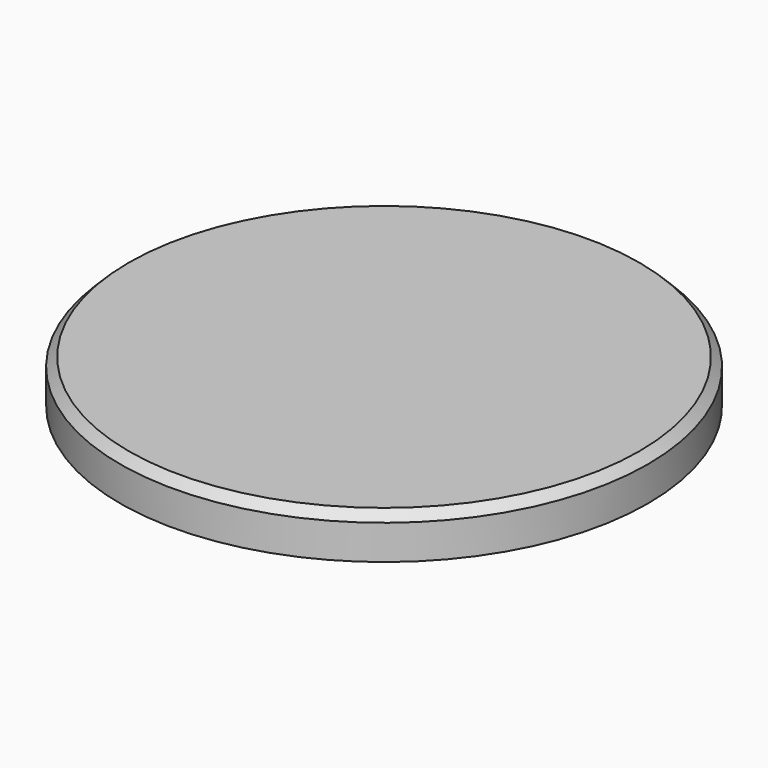
from build123d import *

# Parameters (mm, degrees)
F0_R     = 30.5456119657
F1_DEPTH = 5
F2_SIZE  = 1


# Not quite as in the source:
# - the program builds the solid bodies; features that only make, move or delete a surface that nothing else refers to are left out


with BuildPart() as f1:
    # F0 (on Top) → F1 (new body)
    with BuildSketch(Plane.XY):
        Circle(F0_R)
    extrude(amount=F1_DEPTH)

    # F2
    f2_edges = [f1.edges().sort_by_distance(p)[0] for p in [
        (-30.545612, 0, 5),
    ]]
    chamfer(f2_edges, length=F2_SIZE)


solid = f1.part
